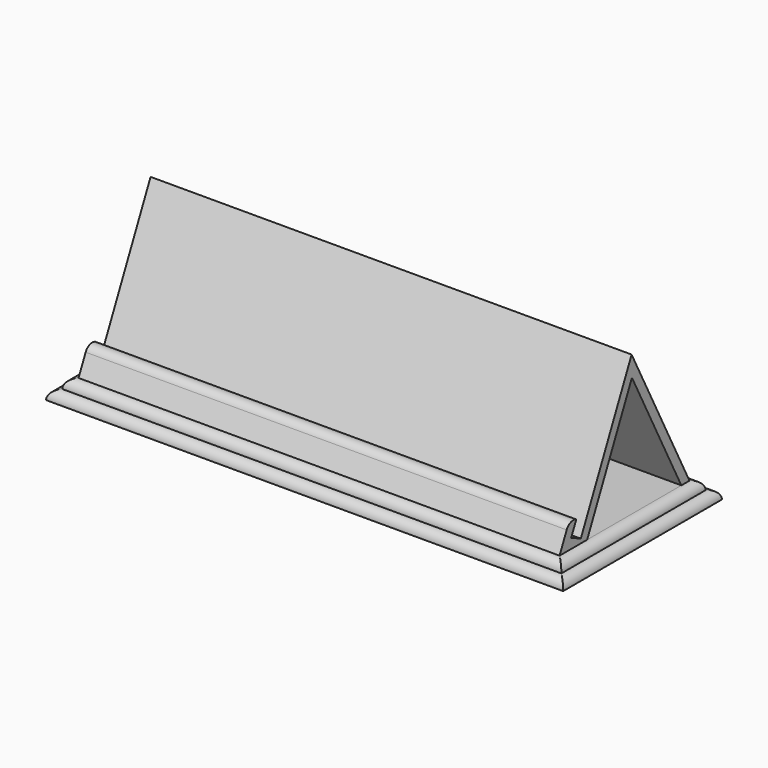
from build123d import *

# Parameters (mm, degrees)
F1_DEPTH = 101.6
F2_DEPTH = 105.41
F3_R     = 3.80999
F4_R     = 3.80999
F5_DEPTH = 109.22
F6_R     = 3.80999


# Not quite as in the source:
# - a fillet or chamfer is up to 0.001 mm smaller than in the source, because OpenCascade refuses the exact size


with BuildPart() as f1:
    # F0 (on Right) → F1 (new body, symmetric)
    with BuildSketch(Plane.YZ):
        Polygon((-28.9227480759, 13.4151088954), (-34.29, 1.905), (-19.7165844463, 1.905), (3.9163465702, 52.5859841168), (30.004847431, 1.905), (34.29, 1.905), (3.7473661652, 61.2388325007), (-23.0888934554, 3.6882880238), (-28.1533413693, 6.0498788705), (-25.4697154073, 11.8049333181), align=None)
    extrude(amount=F1_DEPTH, both=True)

    # F0 (on Right) → F2 (join, symmetric)
    with BuildSketch(Plane.YZ):
        Polygon((-38.1, 1.905), (-38.1, -1.905), (38.1, -1.905), (38.1, 1.905), (34.29, 1.905), (30.004847431, 1.905), (-19.7165844463, 1.905), (-34.29, 1.905), align=None)
    extrude(amount=F2_DEPTH, both=True)

    # F3 (radius 3.81 in the source; OpenCascade refuses exactly that, so slightly less here)
    f3_edges = [f1.edges().sort_by_distance(p)[0] for p in [
        (-105.41, 0, 1.905),
        (0, -38.1, 1.905),
        (0, 38.1, 1.905),
        (105.41, 0, 1.905),
    ]]
    fillet(f3_edges, radius=F3_R)

    # F4 (radius 3.81 in the source; OpenCascade refuses exactly that, so slightly less here)
    f4_edges = [f1.edges().sort_by_distance(p)[0] for p in [
        (0, -28.922748, 13.415109),
    ]]
    fillet(f4_edges, radius=F4_R)

    # F0 (on Right) → F5 (join, symmetric)
    with BuildSketch(Plane.YZ):
        Polygon((38.1, -1.905), (-38.1, -1.905), (-41.91, -1.905), (-41.91, -5.715), (41.91, -5.715), (41.91, -1.905), align=None)
    extrude(amount=F5_DEPTH, both=True)

    # F6 (radius 3.81 in the source; OpenCascade refuses exactly that, so slightly less here)
    f6_edges = [f1.edges().sort_by_distance(p)[0] for p in [
        (-109.22, 0, -1.905),
        (0, 41.91, -1.905),
        (109.22, 0, -1.905),
        (0, -41.91, -1.905),
    ]]
    fillet(f6_edges, radius=F6_R)


solid = f1.part
